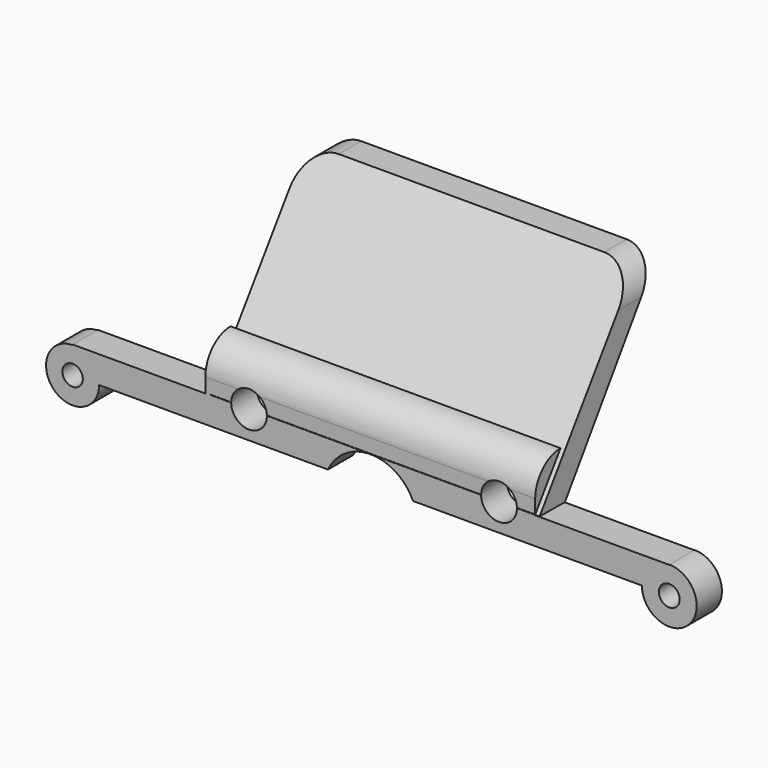
from build123d import *

# Parameters (mm, degrees)
F0_R     = 1.6132793462
F0_R_2   = 1.6452292319
F1_DEPTH = 5
F4_DEPTH = 52
F5_W     = 5.1189595833
F5_H     = 18.4771826025
F6_DEPTH = 78.0283830646
F7_R     = 4.99999
F8_R     = 2.8294209196
F8_R_2   = 2.8212759524
F8_R_3   = 7.3886605842
F9_DEPTH = 25


# Not quite as in the source:
# - a fillet or chamfer is up to 0.001 mm smaller than in the source, because OpenCascade refuses the exact size


with BuildPart() as f1:
    # F0 (on Front) → F1 (new body)
    with BuildSketch(Plane.XZ):
        with BuildLine():
            Line((-40.6402352101, -8.6803976446), (45.1620352523, -8.6803976446))
            ThreePointArc((45.1620352523, -8.6803976446), (52.5455844959, -11.7387638798), (49.4872182608, -4.3552146362))
            Line((49.4872182608, -4.3552146362), (49.4872182608, -4.395077005))
            Line((49.4872182608, -4.395077005), (28.2908082008, -4.395077005))
            Line((28.2908082008, -4.395077005), (28.2908082008, 21.208807826))
            Line((28.2908082008, 21.208807826), (-23.8502826542, 21.208807826))
            Line((-23.8502826542, 21.208807826), (-23.8502826542, -4.395077005))
            Line((-23.8502826542, -4.395077005), (-44.8338091373, -4.395077005))
            Line((-44.8338091373, -4.395077005), (-44.8338091373, -4.4868237174))
            ThreePointArc((-44.8338091373, -4.4868237174), (-47.7991136987, -11.645702206), (-40.6402352101, -8.6803976446))
        make_face()
        with Locations((-44.8338091373, -8.6803976446)):
            Circle(F0_R, mode=Mode.SUBTRACT)
        with Locations((49.4872182608, -8.6803976446)):
            Circle(F0_R_2, mode=Mode.SUBTRACT)
    extrude(amount=F1_DEPTH)

    # F3 (on offset) → F4 (join)
    with BuildSketch(Plane.YZ.offset(29)):
        Polygon((14.035618864, 23.0911467224), (-5.0185876898, -4.3173860759), (0, -4.3494757265), (18.4650830925, 23.0911467224), align=None)
    extrude(amount=-F4_DEPTH)

    # F5 (on offset) → F6 (cut, through all)
    with BuildSketch(Plane.YZ.offset(29)):
        with Locations((-2.5594797917, 12.1628475608)):
            Rectangle(F5_W, F5_H)
    extrude(amount=-F6_DEPTH, mode=Mode.SUBTRACT)

    # F7 (radius 5 in the source; OpenCascade refuses exactly that, so slightly less here)
    f7_edges = [f1.edges().sort_by_distance(p)[0] for p in [
        (-23, 16.250351, 23.091147),
        (29, 16.250351, 23.091147),
        (2.220263, -5, 2.924256),
    ]]
    fillet(f7_edges, radius=F7_R)

    # F8 (on face) → F9 (cut)
    with BuildSketch(Plane(origin=(0, 0, 0), x_dir=(-1, 0, 0), z_dir=(0, 1, 0))):
        with Locations((-22.5741807371, -4.3494757265)):
            Circle(F8_R)
        with Locations((16.9429704547, -4.3494757265)):
            Circle(F8_R_2)
        with Locations((-2.2609000211, -11.7509029806)):
            Circle(F8_R_3)
    extrude(amount=-F9_DEPTH, mode=Mode.SUBTRACT)


solid = f1.part
